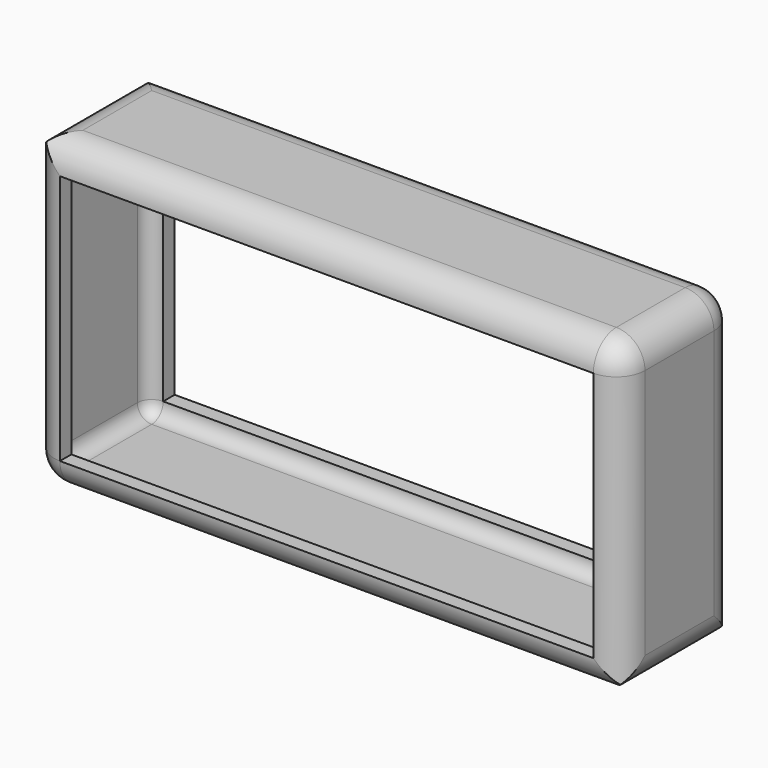
from build123d import *

# Parameters (mm, degrees)
F0_W         = 104.5865043998
F0_H         = 54.5481517911
F1_DEPTH     = 12.7
F2_R         = 5.08
F3_T1_DEPTH  = 57.0881517911
F3_T3_DEPTH  = 15.24
F3_T5_DEPTH  = 107.1265043998
F3_S9_W      = 5.1816
F3_S9_H      = 5.1816
F3_T10_DEPTH = 5.1816
F3_S15_W     = 5.1816
F3_S15_H     = 5.1816
F3_T16_DEPTH = 5.1816
F4_T         = -2.54


# Not quite as in the source:
# - a fillet or chamfer that OpenCascade refuses, or shapes differently, is made with other operations: its cross-section is extruded or revolved along the edge and cut away or added
# - a shell that OpenCascade refuses in one call is made with other operations: the cavity is built on its own and cut out


with BuildPart() as f1:
    # F0 (on Front) → F1 (new body, symmetric)
    with BuildSketch(Plane.XZ):
        Rectangle(F0_W, F0_H)
    extrude(amount=F1_DEPTH, both=True)

    # F2
    f2_edges = [f1.edges().sort_by_distance(p)[0] for p in [
        (52.293252, 0, 27.274076),
        (0, 12.7, 27.274076),
        (-52.293252, 0, 27.274076),
        (0, -12.7, 27.274076),
        (52.293252, 0, -27.274076),
        (52.293252, 12.7, 0),
        (52.293252, -12.7, 0),
    ]]
    fillet(f2_edges, radius=F2_R)

    # F3: fillet of radius 5.08 on 7 edges, made by hand

    # F3_s2 → F3_t1 (cut)
    with BuildSketch(Plane.XY.offset(-22.1940758955)):
        with BuildLine():
            ThreePointArc((-47.2132521999, 12.7), (-50.8053546483, 11.2121024484), (-52.2932521999, 7.62))
            Line((-52.2932521999, 7.62), (-52.2932521999, 12.7))
            Line((-52.2932521999, 12.7), (-47.2132521999, 12.7))
        make_face()
        with BuildLine():
            ThreePointArc((-52.2932521999, -7.62), (-50.8053546483, -11.2121024484), (-47.2132521999, -12.7))
            Line((-47.2132521999, -12.7), (-52.2932521999, -12.7))
            Line((-52.2932521999, -12.7), (-52.2932521999, -7.62))
        make_face()
    extrude(amount=F3_T1_DEPTH, mode=Mode.SUBTRACT)

    # F3_s4 → F3_t3 (cut)
    with BuildSketch(Plane.XZ.offset(-7.62)):
        with BuildLine():
            ThreePointArc((-47.2132521999, -27.2740758955), (-50.8053546483, -25.786178344), (-52.2932521999, -22.1940758955))
            Line((-52.2932521999, -22.1940758955), (-52.2932521999, -27.2740758955))
            Line((-52.2932521999, -27.2740758955), (-47.2132521999, -27.2740758955))
        make_face()
    extrude(amount=F3_T3_DEPTH, mode=Mode.SUBTRACT)

    # F3_s6 → F3_t5 (cut)
    with BuildSketch(Plane.YZ.offset(-47.2132521999)):
        with BuildLine():
            ThreePointArc((7.62, -27.2740758955), (11.2121024484, -25.786178344), (12.7, -22.1940758955))
            Line((12.7, -22.1940758955), (12.7, -27.2740758955))
            Line((12.7, -27.2740758955), (7.62, -27.2740758955))
        make_face()
        with BuildLine():
            ThreePointArc((-7.62, -27.2740758955), (-11.2121024484, -25.786178344), (-12.7, -22.1940758955))
            Line((-12.7, -22.1940758955), (-12.7, -27.2740758955))
            Line((-12.7, -27.2740758955), (-7.62, -27.2740758955))
        make_face()
    extrude(amount=F3_T5_DEPTH, mode=Mode.SUBTRACT)


with BuildPart() as f3_tool8:
    # F3_s9 → F3_t10 (new body)
    with BuildSketch(Plane.XY.offset(-22.1940758955)):
        with Locations((-49.8040521999, 10.2108)):
            Rectangle(F3_S9_W, F3_S9_H)
    extrude(amount=-F3_T10_DEPTH)

    # F3_s11 → F3_t12 (revolve, cut)
    with BuildSketch(Plane(origin=(-47.2132521999, 7.62, -22.1940758955), x_dir=(0.7071067812, -0.7071067812, 0), z_dir=(0.7071067812, 0.7071067812, 0))):
        with BuildLine():
            ThreePointArc((0, -5.08), (5.08, 0), (0, 5.08))
            Line((0, 5.08), (0, -5.08))
        make_face()
    revolve(axis=Axis((-47.2132521999, 7.62, -22.1940758955), (0, 0, -1)), mode=Mode.SUBTRACT)


with BuildPart() as f1_1:
    add(f1.part)

    # F3_t7: cut F3_tool8
    add(f3_tool8.part, mode=Mode.SUBTRACT)


with BuildPart() as f3_tool14:
    # F3_s15 → F3_t16 (new body)
    with BuildSketch(Plane.XY.offset(-22.1940758955)):
        with Locations((-49.8040521999, -10.2108)):
            Rectangle(F3_S15_W, F3_S15_H)
    extrude(amount=-F3_T16_DEPTH)

    # F3_s17 → F3_t18 (revolve, cut)
    with BuildSketch(Plane(origin=(-47.2132521999, -7.62, -22.1940758955), x_dir=(0.7071067812, 0.7071067812, 0), z_dir=(-0.7071067812, 0.7071067812, 0))):
        with BuildLine():
            ThreePointArc((0, -5.08), (5.08, 0), (0, 5.08))
            Line((0, 5.08), (0, -5.08))
        make_face()
    revolve(axis=Axis((-47.2132521999, -7.62, -22.1940758955), (0, 0, -1)), mode=Mode.SUBTRACT)


with BuildPart() as f1_2:
    add(f1_1.part)

    # F3_t13: cut F3_tool14
    add(f3_tool14.part, mode=Mode.SUBTRACT)

    # F4: a shell. OpenCascade refuses it in one call, so the cavity is built on its own and cut out:
    # the body offset inwards by the wall thickness, plus a prism from it out through each open face.
    f4_core = offset(f1_2.part, amount=F4_T, mode=Mode.PRIVATE)
    f4_exits = [f4_core.faces().sort_by_distance(p)[0] for p in [
        (0, -10.16, 0),
        (0, 10.16, 0),
    ]]
    add(f4_core, mode=Mode.SUBTRACT)
    extrude(f4_exits, amount=-F4_T, mode=Mode.SUBTRACT)


solid = f1_2.part
